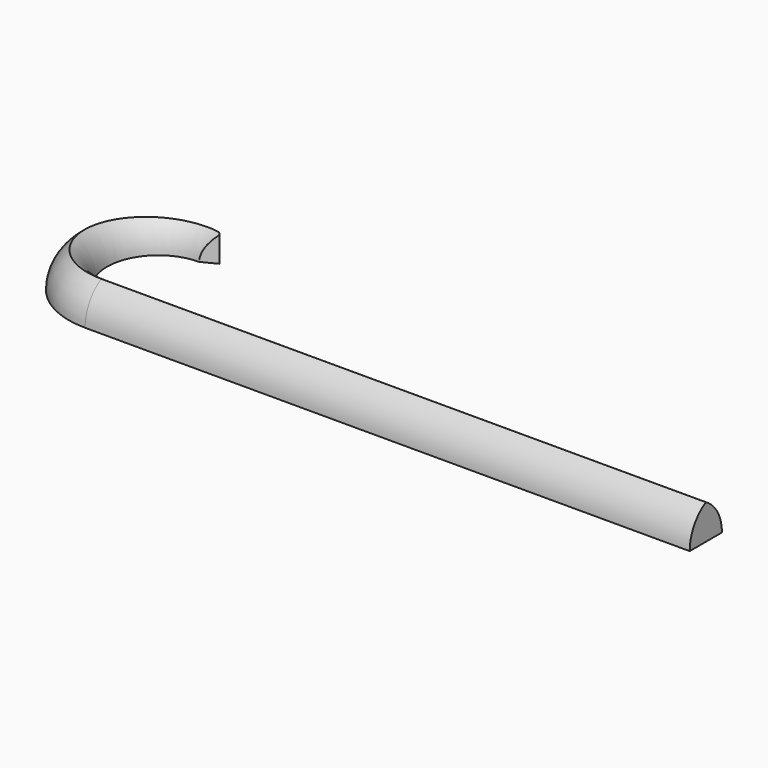
from build123d import *

# Parameters (mm, degrees)
F1_DEPTH    = 5.08
F0_W        = 76.2
F0_H        = 5.08
F2_DEPTH    = 5.08
F3_T1_DEPTH = 88.9
F3_T4_ANGLE = 251.0303843405
F3_T6_ANGLE = 292.9828431402


# Not quite as in the source:
# - a fillet or chamfer that OpenCascade refuses, or shapes differently, is made with other operations: its cross-section is extruded or revolved along the edge and cut away or added


with BuildPart() as f1:
    # F0 (on Top) → F1 (new body)
    with BuildSketch(Plane.XY):
        with BuildLine():
            Line((-38.1, -2.54), (-38.1, 2.54))
            ThreePointArc((-38.1, 2.54), (-44.5507724238, 8.9907724238), (-38.1, 15.4415448477))
            Line((-38.1, 15.4415448477), (-36.2862832844, 16.3751454373))
            Line((-36.2862832844, 16.3751454373), (-38.1, 17.9815448477))
            ThreePointArc((-38.1, 17.9815448477), (-48.3607724238, 7.7207724238), (-38.1, -2.54))
        make_face()
    extrude(amount=F1_DEPTH)

    # F0 (on Top) → F2 (join)
    with BuildSketch(Plane.XY):
        Rectangle(F0_W, F0_H)
    extrude(amount=F2_DEPTH)

    # F3: fillet of radius 5.08 on 2 edges, made by hand

    # F3_s2 → F3_t1 (cut)
    with BuildSketch(Plane.YZ.offset(-38.1)):
        with BuildLine():
            ThreePointArc((-2.54, 5.08), (1.0521024484, 3.5921024484), (2.54, 0))
            Line((2.54, 0), (2.54, 5.08))
            Line((2.54, 5.08), (-2.54, 5.08))
        make_face()
        with BuildLine():
            ThreePointArc((-2.54, 0), (-1.0521024484, 3.5921024484), (2.54, 5.08))
            Line((2.54, 5.08), (-2.54, 5.08))
            Line((-2.54, 5.08), (-2.54, 0))
        make_face()
    extrude(amount=F3_T1_DEPTH, mode=Mode.SUBTRACT)

    # F3_s3 → F3_t4 (revolve, cut)
    with BuildSketch(Plane(origin=(-6.3994276616, 18.6173540989, 0), x_dir=(0, 0, 1), z_dir=(0.3250666938, -0.9456910936, 0))):
        with BuildLine():
            ThreePointArc((0, 23.2602922785), (3.5921024484, 24.7481898301), (5.08, 28.3402922785))
            Line((5.08, 28.3402922785), (5.08, 23.2602922785))
            Line((5.08, 23.2602922785), (0, 23.2602922785))
        make_face()
    revolve(axis=Axis((-38.1, 7.7207724238, 5.08), (0, 0, 1)), revolution_arc=F3_T4_ANGLE, mode=Mode.SUBTRACT)

    # F3_s5 → F3_t6 (revolve, cut)
    with BuildSketch(Plane.YZ.offset(-38.1)):
        with BuildLine():
            ThreePointArc((-2.54, 5.08), (1.0521024484, 3.5921024484), (2.54, 0))
            Line((2.54, 0), (2.54, 5.08))
            Line((2.54, 5.08), (-2.54, 5.08))
        make_face()
    revolve(axis=Axis((-38.1, 8.9907724238, 5.08), (0, 0, -1)), revolution_arc=F3_T6_ANGLE, mode=Mode.SUBTRACT)


solid = f1.part
